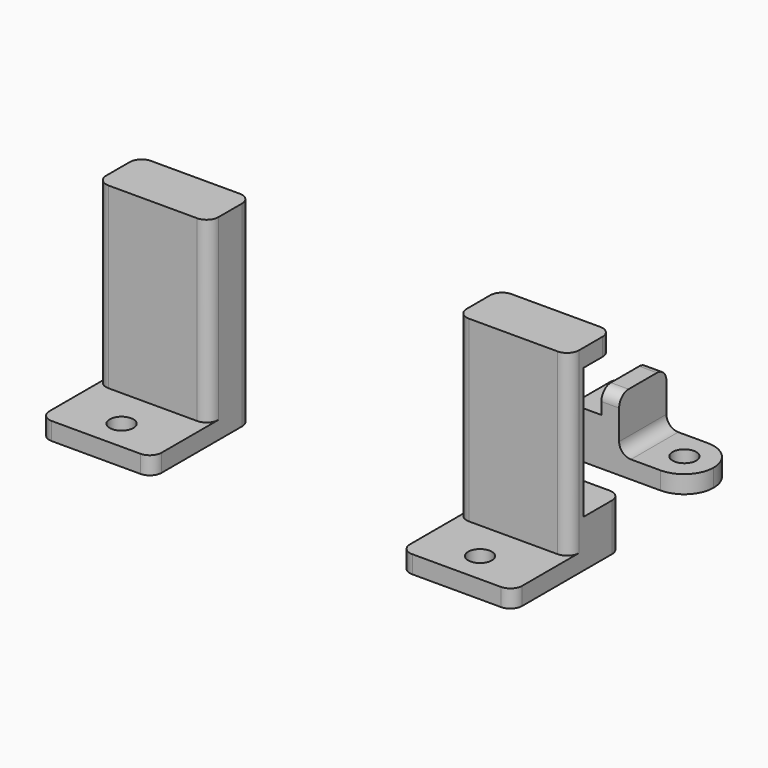
from build123d import *

# Parameters (mm, degrees)
F0_W      = 16
F0_H      = 8
F1_DEPTH  = 8
F2_W      = 16
F2_H      = 3
F3_DEPTH  = 33.2
F4_W      = 19
F4_H      = 3
F5_DEPTH  = 12
F6_R      = 2
F7_DEPTH  = 3
F8_W      = 16
F8_H      = 3
F9_DEPTH  = 6
F10_R     = 1.99999
F13_W     = 8
F13_H     = 10
F14_DEPTH = 8
F15_W     = 10
F15_H     = 3
F16_DEPTH = 12
F17_W     = 3
F17_H     = 10
F18_DEPTH = 4
F19_R     = 2
F20_DEPTH = 3
F21_R     = 4.99999
F22_R     = 2


# Not quite as in the source:
# - a fillet or chamfer is up to 0.001 mm smaller than in the source, because OpenCascade refuses the exact size


with BuildPart() as f1:
    # F0 (on Top) → F1 (new body)
    with BuildSketch(Plane.XY):
        with Locations((-8, 4)):
            Rectangle(F0_W, F0_H)
    extrude(amount=F1_DEPTH)

    # F2 (on Top) → F3 (join)
    with BuildSketch(Plane.XY):
        with Locations((-8, -1.5)):
            Rectangle(F2_W, F2_H)
        Polygon((0, 6), (0, 0), (0, -3), (3, -3), (3, 6), align=None)
    extrude(amount=F3_DEPTH)

    # F4 (on face) → F5 (join)
    with BuildSketch(Plane.XZ.offset(3)):
        with Locations((-6.5, 1.5)):
            Rectangle(F4_W, F4_H)
    extrude(amount=F5_DEPTH)

    # F6 (on face) → F7 (cut, through all)
    with BuildSketch(Plane.XY.offset(3)):
        with Locations((-6.3249543309, -9.8292976618)):
            Circle(F6_R)
    extrude(amount=-F7_DEPTH, mode=Mode.SUBTRACT)

    # F8 (on face) → F9 (join)
    with BuildSketch(Plane(origin=(0, 0, 0), x_dir=(-1, 0, 0), z_dir=(0, 1, 0))):
        with Locations((8, 31.7)):
            Rectangle(F8_W, F8_H)
    extrude(amount=F9_DEPTH)

    # F10 (radius 2 in the source; OpenCascade refuses exactly that, so slightly less here)
    f10_edges = [f1.edges().sort_by_distance(p)[0] for p in [
        (-16, 6, 31.7),
        (-16, 8, 4),
        (0, 8, 4),
        (3, 6, 16.6),
        (3, -15, 1.5),
        (3, -3, 18.1),
        (-16, -3, 18.1),
        (-16, -15, 1.5),
    ]]
    fillet(f10_edges, radius=F10_R)


with BuildPart() as f12_1:
    # F12: instance of F1
    add(f1.part.mirror(Plane.YZ.offset(24)))


with BuildPart() as f14:
    # F13 (on Top) → F14 (new body)
    with BuildSketch(Plane.XY):
        with Locations((46.6220968366, 29.2166761309)):
            Rectangle(F13_W, F13_H)
    extrude(amount=F14_DEPTH)

    # F15 (on face) → F16 (join)
    with BuildSketch(Plane.YZ.offset(50.6220968366)):
        with Locations((29.2166761309, 1.5)):
            Rectangle(F15_W, F15_H)
    extrude(amount=F16_DEPTH)

    # F17 (on face) → F18 (join)
    with BuildSketch(Plane.XY.offset(8)):
        with Locations((49.1220968366, 29.2166761309)):
            Rectangle(F17_W, F17_H)
    extrude(amount=F18_DEPTH)

    # F19 (on face) → F20 (cut, through all)
    with BuildSketch(Plane.XY.offset(3)):
        with Locations((57.5763136148, 29.331497848)):
            Circle(F19_R)
    extrude(amount=-F20_DEPTH, mode=Mode.SUBTRACT)

    # F21 (radius 5 in the source; OpenCascade refuses exactly that, so slightly less here)
    f21_edges = [f14.edges().sort_by_distance(p)[0] for p in [
        (62.622097, 34.216676, 1.5),
        (62.622097, 24.216676, 1.5),
    ]]
    fillet(f21_edges, radius=F21_R)

    # F22
    f22_edges = [f14.edges().sort_by_distance(p)[0] for p in [
        (50.622097, 29.216676, 3),
        (49.122097, 34.216676, 12),
        (49.122097, 24.216676, 12),
        (42.622097, 34.216676, 4),
        (42.622097, 24.216676, 4),
    ]]
    fillet(f22_edges, radius=F22_R)


solid = Compound([f1.part, f12_1.part, f14.part])
